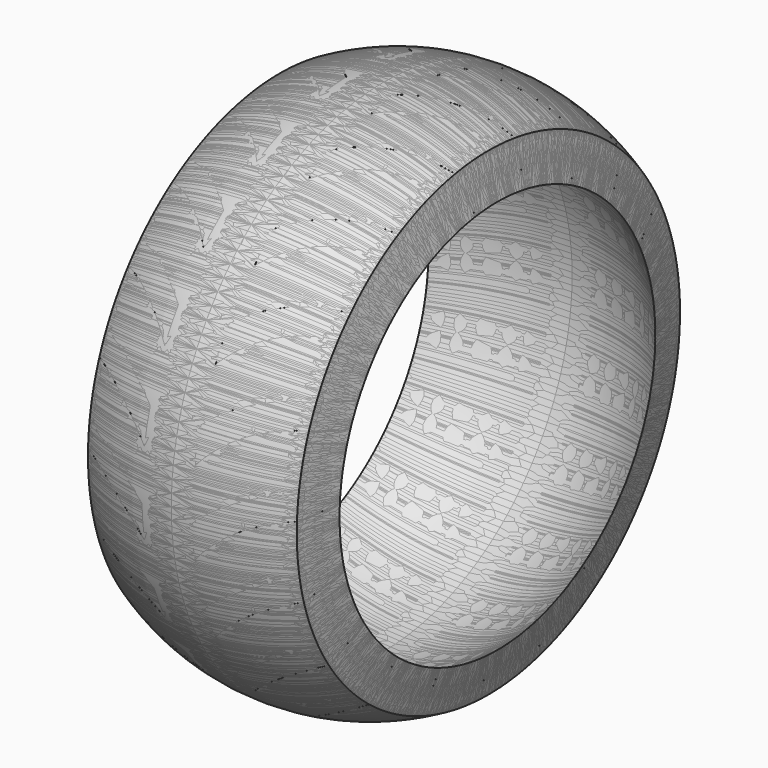
from build123d import *

# Parameters (mm, degrees)
F4_DEPTH = 70.612
F5_COUNT = 20


# Not quite as in the source:
# - ends of sketch curves that miss each other by under 0.0002 mm in the source are joined
# - the dataset's text gives a spline's control points without its knots; the knots are read off the source's solid


with BuildPart() as f1:
    # F0 (on Front) → F1 (revolve)
    with BuildSketch(Plane.XZ):
        with BuildLine():
            ThreePointArc((-18.729841673, 32.7820238305), (-9.8237527413, 37.4340040502), (0.0919083894, 39.0585053166))
            ThreePointArc((0.0919083894, 39.0585053166), (10.0075695201, 37.4340040502), (18.9136584518, 32.7820238305))
            Line((18.9136584518, 32.7820238305), (17.4176339561, 39.7441881909))
            ThreePointArc((17.4176339561, 39.7441881909), (9.0262708039, 43.0118086206), (0.0919083894, 44.1385237894))
            ThreePointArc((0.0919083894, 44.1385237894), (-8.8424540251, 43.0118086206), (-17.2338171773, 39.7441881909))
            Line((-17.2338171773, 39.7441881909), (-18.729841673, 32.7820238305))
        make_face()
    revolve(axis=Axis((2.7360580862, 0, 0), (1, 0, 0)))

    # F3 (on offset) → F4 (cut)
    with BuildSketch(Plane.XZ.offset(76.2)):
        with BuildLine():
            add(Edge.make_bspline(
                [(-23.8198616895, 5.7528143142), (-17.5698088787, 6.0817643781), (-10.8331610484, 4.0608614944), (-5.0887438734, -1.3304929032)],
                knots=[0, 0, 0, 0, 22.1571793055, 22.1571793055, 22.1571793055, 22.1571793055], degree=3))
            Line((-23.8198616895, 5.7528143142), (-23.6196125863, 1.9480803818))
            add(Edge.make_bspline(
                [(-23.6196125863, 1.9480803818), (-21.3060253639, 2.0698480992), (-17.7297466947, 1.6829007424), (-13.0253372983, -0.1906570227), (-9.5789126742, -2.3491849401), (-6.948673347, -4.7392742599), (-5.4888893533, -6.4324495982), (-5.0887086474, -6.9284101766)],
                knots=[0, 0, 0, 0, 0.25, 0.375, 0.5, 0.625, 0.6732153409, 0.6732153409, 0.6732153409, 0.6732153409], degree=3))
            Line((-5.0887086474, -6.9284101766), (-5.0887438734, -1.3304929032))
        make_face()
        with BuildLine():
            add(Edge.make_bspline(
                [(22.2290589121, 5.7528143142), (15.9790061011, 6.0817643781), (9.2423582705, 4.0608614943), (3.4979410953, -1.3304929038)],
                knots=[0, 0, 0, 0, 22.1571793064, 22.1571793064, 22.1571793064, 22.1571793064], degree=3))
            Line((3.4979410953, -1.3304929038), (3.4979410802, -6.9284385845))
            ThreePointArc((3.4979410802, -6.9284385845), (4.7499874456, -5.4741516418), (6.1016775203, -4.1119825793))
            add(Edge.make_bspline(
                [(22.0288098089, 1.9480803818), (19.7152225866, 2.0698480992), (16.1389439173, 1.6829007424), (11.434534521, -0.1906570227), (8.4787418077, -2.0418975939), (6.7290527758, -3.5228712713), (6.1016775203, -4.1119825793)],
                knots=[0, 0, 0, 0, 0.25, 0.375, 0.5, 0.5716151195, 0.5716151195, 0.5716151195, 0.5716151195], degree=3))
            Line((22.0288098089, 1.9480803818), (22.2290589121, 5.7528143142))
        make_face()
    extrude(amount=-F4_DEPTH, mode=Mode.SUBTRACT)


with BuildPart() as f5_1:
    # F5: instance of F1
    add(f1.part.rotate(Axis((-17.2338171773, 0, 0), (-1, 0, 0)), 1 * 360 / F5_COUNT))


with BuildPart() as f5_2:
    # F5: instance of F1
    add(f1.part.rotate(Axis((-17.2338171773, 0, 0), (-1, 0, 0)), 2 * 360 / F5_COUNT))


with BuildPart() as f5_3:
    # F5: instance of F1
    add(f1.part.rotate(Axis((-17.2338171773, 0, 0), (-1, 0, 0)), 3 * 360 / F5_COUNT))


with BuildPart() as f5_4:
    # F5: instance of F1
    add(f1.part.rotate(Axis((-17.2338171773, 0, 0), (-1, 0, 0)), 4 * 360 / F5_COUNT))


with BuildPart() as f5_5:
    # F5: instance of F1
    add(f1.part.rotate(Axis((-17.2338171773, 0, 0), (-1, 0, 0)), 5 * 360 / F5_COUNT))


with BuildPart() as f5_6:
    # F5: instance of F1
    add(f1.part.rotate(Axis((-17.2338171773, 0, 0), (-1, 0, 0)), 6 * 360 / F5_COUNT))


with BuildPart() as f5_7:
    # F5: instance of F1
    add(f1.part.rotate(Axis((-17.2338171773, 0, 0), (-1, 0, 0)), 7 * 360 / F5_COUNT))


with BuildPart() as f5_8:
    # F5: instance of F1
    add(f1.part.rotate(Axis((-17.2338171773, 0, 0), (-1, 0, 0)), 8 * 360 / F5_COUNT))


with BuildPart() as f5_9:
    # F5: instance of F1
    add(f1.part.rotate(Axis((-17.2338171773, 0, 0), (-1, 0, 0)), 9 * 360 / F5_COUNT))


with BuildPart() as f5_10:
    # F5: instance of F1
    add(f1.part.rotate(Axis((-17.2338171773, 0, 0), (-1, 0, 0)), 10 * 360 / F5_COUNT))


with BuildPart() as f5_11:
    # F5: instance of F1
    add(f1.part.rotate(Axis((-17.2338171773, 0, 0), (-1, 0, 0)), 11 * 360 / F5_COUNT))


with BuildPart() as f5_12:
    # F5: instance of F1
    add(f1.part.rotate(Axis((-17.2338171773, 0, 0), (-1, 0, 0)), 12 * 360 / F5_COUNT))


with BuildPart() as f5_13:
    # F5: instance of F1
    add(f1.part.rotate(Axis((-17.2338171773, 0, 0), (-1, 0, 0)), 13 * 360 / F5_COUNT))


with BuildPart() as f5_14:
    # F5: instance of F1
    add(f1.part.rotate(Axis((-17.2338171773, 0, 0), (-1, 0, 0)), 14 * 360 / F5_COUNT))


with BuildPart() as f5_15:
    # F5: instance of F1
    add(f1.part.rotate(Axis((-17.2338171773, 0, 0), (-1, 0, 0)), 15 * 360 / F5_COUNT))


with BuildPart() as f5_16:
    # F5: instance of F1
    add(f1.part.rotate(Axis((-17.2338171773, 0, 0), (-1, 0, 0)), 16 * 360 / F5_COUNT))


with BuildPart() as f5_17:
    # F5: instance of F1
    add(f1.part.rotate(Axis((-17.2338171773, 0, 0), (-1, 0, 0)), 17 * 360 / F5_COUNT))


with BuildPart() as f5_18:
    # F5: instance of F1
    add(f1.part.rotate(Axis((-17.2338171773, 0, 0), (-1, 0, 0)), 18 * 360 / F5_COUNT))


with BuildPart() as f5_19:
    # F5: instance of F1
    add(f1.part.rotate(Axis((-17.2338171773, 0, 0), (-1, 0, 0)), 19 * 360 / F5_COUNT))


solid = Compound([f1.part, f5_1.part, f5_2.part, f5_3.part, f5_4.part, f5_5.part, f5_6.part, f5_7.part, f5_8.part, f5_9.part, f5_10.part, f5_11.part, f5_12.part, f5_13.part, f5_14.part, f5_15.part, f5_16.part, f5_17.part, f5_18.part, f5_19.part])
